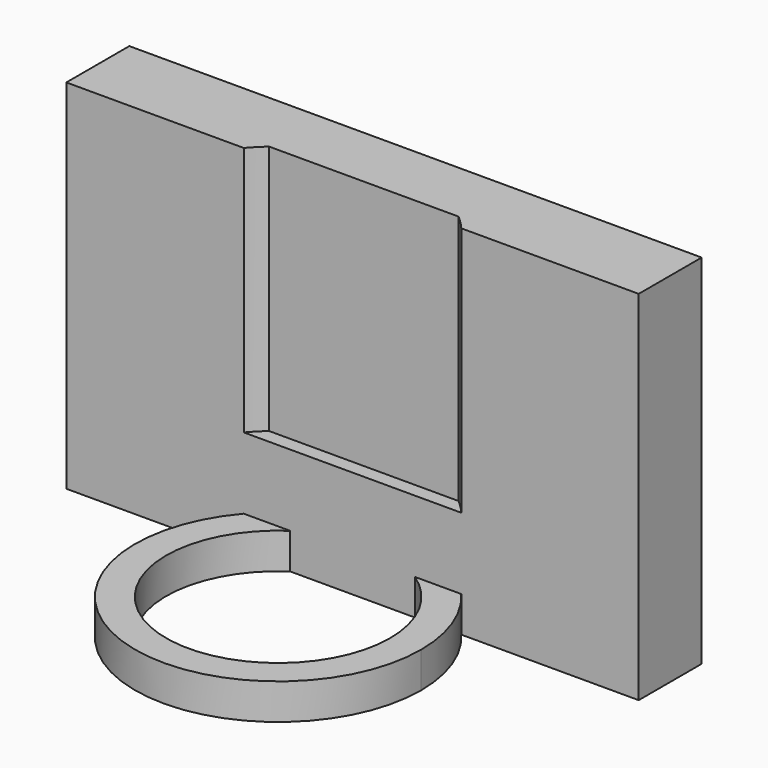
from build123d import *

# Parameters (mm, degrees)
F0_R     = 4.75
F1_DEPTH = 6
F2_R     = 4.75
F3_DEPTH = 11
F5_DEPTH = 5
F7_DEPTH = 35


with BuildPart() as f1:
    # F0 (on Front) → F1 (new body)
    with BuildSketch(Plane.XZ):
        with Locations((-27, 0)):
            Circle(F0_R)
    extrude(amount=F1_DEPTH)


with BuildPart() as f1b:
    # F0 (on Front) → F1, piece 2 (new body)
    with BuildSketch(Plane.XZ):
        with Locations((27, 0)):
            Circle(F0_R)
    extrude(amount=F1_DEPTH)


with BuildPart() as f3:
    # F2 (on face) → F3 (new body)
    with BuildSketch(Plane.XZ.offset(6)):
        Polygon((-40, -15), (40, -15), (40, 15), (40, 35), (-40, 35), (-40, 15), align=None)
        with Locations((-27, 0)):
            Circle(F2_R, mode=Mode.SUBTRACT)
        with Locations((-27, 0)):
            Circle(F2_R)
    extrude(amount=F3_DEPTH)

    # F4 (on face) → F5 (join)
    with BuildSketch(Plane(origin=(0, 0, -15), x_dir=(1, 0, 0), z_dir=(0, 0, -1))):
        with BuildLine():
            ThreePointArc((-8.7133518235, 17), (-7.3674467749, 43.8073613706), (15.65, 30))
            ThreePointArc((15.65, 30), (13.8073613706, 22.6325532251), (8.7133518235, 17))
            Line((8.7133518235, 17), (15.1986841536, 17))
            ThreePointArc((15.1986841536, 17), (18.7613123618, 23.0708472044), (20, 30))
            ThreePointArc((20, 30), (-6.9291527956, 48.7613123618), (-15.1986841536, 17))
            Line((-15.1986841536, 17), (-8.7133518235, 17))
        make_face()
        with BuildLine():
            ThreePointArc((8.7133518235, 17), (0, 14.35), (-8.7133518235, 17))
            Line((-8.7133518235, 17), (-15.1986841536, 17))
            ThreePointArc((-15.1986841536, 17), (0, 10), (15.1986841536, 17))
            Line((15.1986841536, 17), (8.7133518235, 17))
        make_face()
    extrude(amount=-F5_DEPTH)

    # F6 (on face) → F7 (cut)
    with BuildSketch(Plane.XY.offset(35)):
        with BuildLine():
            ThreePointArc((-13.25, -15.0187617334), (-14.2587949626, -15.975494083), (-15.1986841536, -17))
            Line((-15.1986841536, -17), (-13.25, -17))
            Line((-13.25, -17), (-13.25, -15.0187617334))
        make_face()
        Polygon((8.7133518235, -17), (13.25, -17), (13.25, -15.0187617334), (-13.25, -15.0187617334), (-13.25, -17), (-8.7133518235, -17), align=None)
        with BuildLine():
            Line((13.25, -17), (15.1986841536, -17))
            ThreePointArc((15.1986841536, -17), (14.2587949626, -15.975494083), (13.25, -15.0187617334))
            Line((13.25, -15.0187617334), (13.25, -17))
        make_face()
    extrude(amount=-F7_DEPTH, mode=Mode.SUBTRACT)


solid = Compound([f1.part, f1b.part, f3.part])
